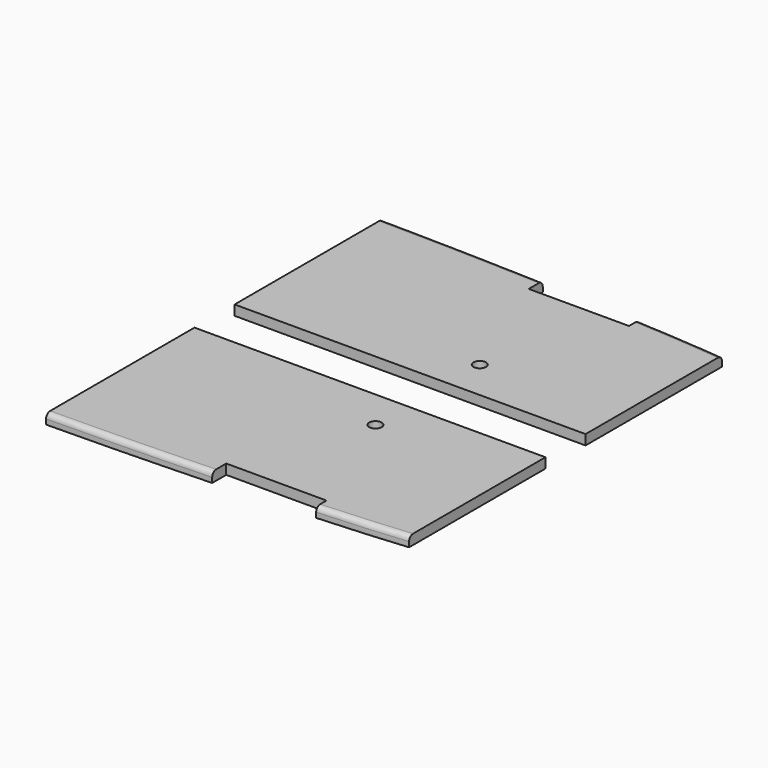
from build123d import *

# Parameters (mm, degrees)
F0_R     = 1.25
F1_DEPTH = 2
F2_DEPTH = 2
F3_R     = 1


# Not quite as in the source:
# - a feature names something its author has since deleted; it is built from what else it names


with BuildPart() as f1:
    # F0 (on Top) → F1 (new body)
    with BuildSketch(Plane.XY):
        with BuildLine():
            Line((0, 37), (0, 0))
            Line((0, 0), (70, 0))
            Line((70, 0), (70, 34))
            add(Edge.make_bspline(
                [(52.5, 35.2891019981), (59.3214395591, 34.9055787176), (65.4248555138, 34.4712498014), (70, 34)],
                knots=[50.2368914557, 50.2368914557, 50.2368914557, 50.2368914557, 70.0642562224, 70.0642562224, 70.0642562224, 70.0642562224], degree=3))
            Line((52.5, 35.2891019981), (52.5, 32.7070827343))
            Line((52.5, 32.7070827343), (32.5, 32.7070827343))
            Line((32.5, 32.7070827343), (32.5, 36.2070827343))
            add(Edge.make_bspline(
                [(0, 37), (8.4901566801, 36.9403682594), (20.460276432, 36.6565820507), (32.5, 36.2070827343)],
                knots=[0, 0, 0, 0, 32.0129533553, 32.0129533553, 32.0129533553, 32.0129533553], degree=3))
        make_face()
        with Locations((42.5, 8)):
            Circle(F0_R, mode=Mode.SUBTRACT)
    extrude(amount=F1_DEPTH)

    # F0 (on Top) → F2 (join)
    with BuildSketch(Plane.XY):
        with BuildLine():
            Line((0, 37), (0, 0))
            Line((0, 0), (70, 0))
            Line((70, 0), (70, 34))
            add(Edge.make_bspline(
                [(52.5, 35.2891019981), (59.3214395591, 34.9055787176), (65.4248555138, 34.4712498014), (70, 34)],
                knots=[50.2368914557, 50.2368914557, 50.2368914557, 50.2368914557, 70.0642562224, 70.0642562224, 70.0642562224, 70.0642562224], degree=3))
            Line((52.5, 35.2891019981), (52.5, 32.7070827343))
            Line((52.5, 32.7070827343), (32.5, 32.7070827343))
            Line((32.5, 32.7070827343), (32.5, 36.2070827343))
            add(Edge.make_bspline(
                [(0, 37), (8.4901566801, 36.9403682594), (20.460276432, 36.6565820507), (32.5, 36.2070827343)],
                knots=[0, 0, 0, 0, 32.0129533553, 32.0129533553, 32.0129533553, 32.0129533553], degree=3))
        make_face()
        with Locations((42.5, 8)):
            Circle(F0_R, mode=Mode.SUBTRACT)
    extrude(amount=F2_DEPTH)

    # F3
    f3_edges = [f1.edges().sort_by_distance(p)[0] for p in [
        (16.252703, 36.716727, 2),
        (61.256993, 34.737622, 2),
    ]]
    fillet(f3_edges, radius=F3_R)


with BuildPart() as f5_1:
    # F5: instance of F1
    add(f1.part.mirror(Plane(origin=(35, -5, 1), x_dir=(1, 0, 0), z_dir=(0, -1, 0))))


solid = Compound([f1.part, f5_1.part])
